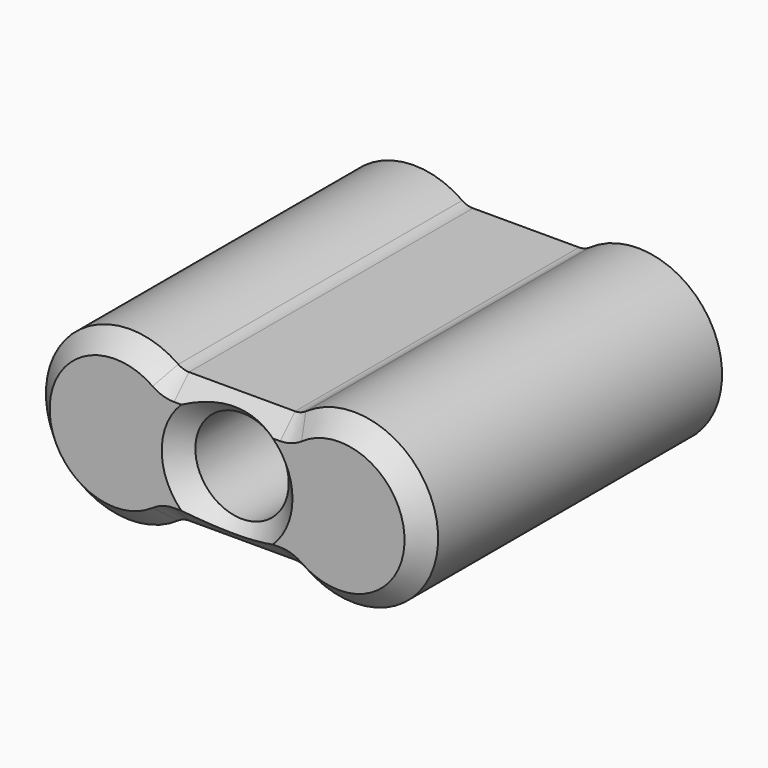
from build123d import *

# Parameters (mm, degrees)
F1_DEPTH     = 101.6
F2_R         = 5.08
F3_R         = 5.08
F4_T1_DEPTH  = 28.8312589727
F4_T4_ANGLE  = 250.1936024552
F4_T6_ANGLE  = 35.0968012276
F4_T8_ANGLE  = 35.0968012276
F4_T10_ANGLE = 35.0968012276
F4_T12_ANGLE = 35.0968012276
F4_T14_ANGLE = 250.1936024552


# Not quite as in the source:
# - a fillet or chamfer that OpenCascade refuses, or shapes differently, is made with other operations: its cross-section is extruded or revolved along the edge and cut away or added


with BuildPart() as f1:
    # F0 (on Front) → F1 (new body)
    with BuildSketch(Plane.XZ):
        with BuildLine():
            Line((16.1115902063, 17.78), (-16.1115902063, 17.78))
            ThreePointArc((-16.1115902063, 17.78), (-53.34, 0), (-16.1115902063, -17.78))
            Line((-16.1115902063, -17.78), (16.1115902063, -17.78))
            ThreePointArc((16.1115902063, -17.78), (53.34, 0), (16.1115902063, 17.78))
        make_face()
        with BuildLine():
            ThreePointArc((-12.7, 0), (0, 12.7), (12.7, 0))
            ThreePointArc((12.7, 0), (0, -12.7), (-12.7, 0))
        make_face(mode=Mode.SUBTRACT)
    extrude(amount=F1_DEPTH)

    # F2
    f2_edges = [f1.edges().sort_by_distance(p)[0] for p in [
        (-16.11159, -50.8, 17.78),
        (16.11159, -50.8, 17.78),
    ]]
    fillet(f2_edges, radius=F2_R)

    # F3
    f3_edges = [f1.edges().sort_by_distance(p)[0] for p in [
        (-16.11159, -50.8, -17.78),
        (16.11159, -50.8, -17.78),
    ]]
    fillet(f3_edges, radius=F3_R)

    # F4: chamfer of 5.08 on 9 edges, made by hand

    # F4_s2 → F4_t1 (cut)
    with BuildSketch(Plane.YZ.offset(-14.4156294863)):
        Polygon((-96.52, -17.78), (-101.6, -12.7), (-101.6, -17.78), align=None)
        Polygon((-96.52, 17.78), (-101.6, 12.7), (-101.6, 17.78), align=None)
    extrude(amount=F4_T1_DEPTH, mode=Mode.SUBTRACT)

    # F4_s3 → F4_t4 (revolve, cut)
    with BuildSketch(Plane(origin=(20.4039669421, 0, -14.3384464089), x_dir=(0, 1, 0), z_dir=(-0.8181818182, 0, 0.5749595746))):
        Polygon((-96.52, 5.3352321669), (-101.6, 0.2552321669), (-101.6, 5.3352321669), align=None)
    revolve(axis=Axis((30.48, -101.6, 0), (0, -1, 0)), revolution_arc=F4_T4_ANGLE, mode=Mode.SUBTRACT)

    # F4_s5 → F4_t6 (revolve, cut)
    with BuildSketch(Plane(origin=(20.4039669421, 0, -14.3384464089), x_dir=(0, 1, 0), z_dir=(0.8181818182, 0, -0.5749595746))):
        Polygon((-96.52, -5.3352321669), (-101.6, -0.2552321669), (-101.6, -5.3352321669), align=None)
    revolve(axis=Axis((14.4156294863, -101.6, -22.86), (0, -1, 0)), revolution_arc=F4_T6_ANGLE, mode=Mode.SUBTRACT)

    # F4_s7 → F4_t8 (revolve, cut)
    with BuildSketch(Plane.YZ.offset(14.4156294863)):
        Polygon((-96.52, 17.78), (-101.6, 12.7), (-101.6, 17.78), align=None)
    revolve(axis=Axis((14.4156294863, -101.6, 22.86), (0, -1, 0)), revolution_arc=F4_T8_ANGLE, mode=Mode.SUBTRACT)

    # F4_s9 → F4_t10 (revolve, cut)
    with BuildSketch(Plane(origin=(-20.4039669421, 0, -14.3384464089), x_dir=(0, 1, 0), z_dir=(-0.8181818182, 0, -0.5749595746))):
        Polygon((-96.52, 5.3352321669), (-101.6, 0.2552321669), (-101.6, 5.3352321669), align=None)
    revolve(axis=Axis((-14.4156294863, -101.6, -22.86), (0, 1, 0)), revolution_arc=F4_T10_ANGLE, mode=Mode.SUBTRACT)

    # F4_s11 → F4_t12 (revolve, cut)
    with BuildSketch(Plane.YZ.offset(-14.4156294863)):
        Polygon((-96.52, 17.78), (-101.6, 12.7), (-101.6, 17.78), align=None)
    revolve(axis=Axis((-14.4156294863, -101.6, 22.86), (0, 1, 0)), revolution_arc=F4_T12_ANGLE, mode=Mode.SUBTRACT)

    # F4_s13 → F4_t14 (revolve, cut)
    with BuildSketch(Plane(origin=(-20.4039669421, 0, 14.3384464089), x_dir=(0, 1, 0), z_dir=(0.8181818182, 0, -0.5749595746))):
        Polygon((-96.52, 5.3352321669), (-101.6, 0.2552321669), (-101.6, 5.3352321669), align=None)
    revolve(axis=Axis((-30.48, -101.6, 0), (0, -1, 0)), revolution_arc=F4_T14_ANGLE, mode=Mode.SUBTRACT)

    # F4_s15 → F4_t16 (revolve, cut)
    with BuildSketch(Plane.XY):
        Polygon((12.7, -96.52), (17.78, -101.6), (12.7, -101.6), align=None)
    revolve(axis=Axis((0, -101.6, 0), (0, -1, 0)), mode=Mode.SUBTRACT)


solid = f1.part
